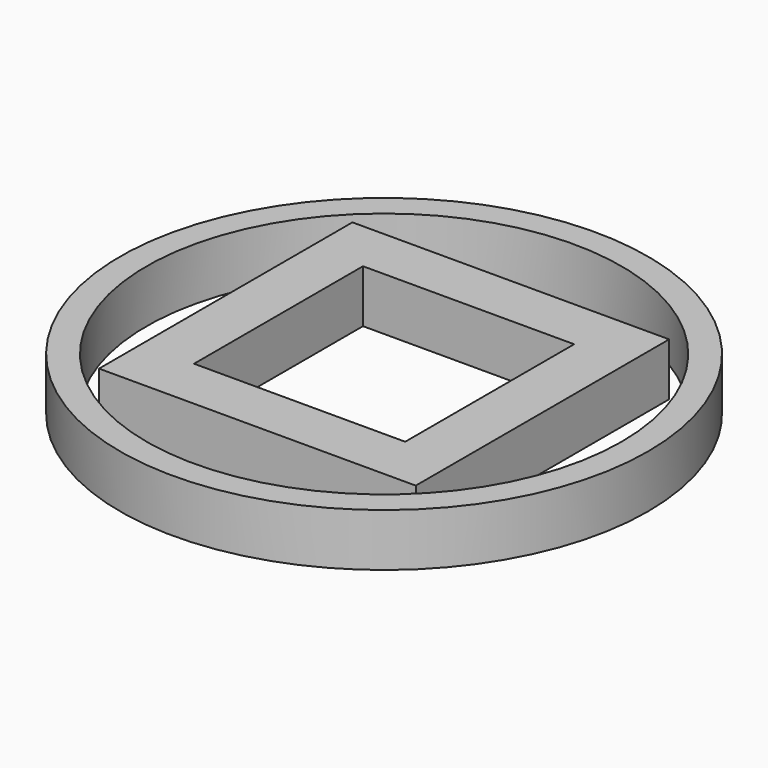
from build123d import *

# Parameters (mm, degrees)
F0_R     = 25
F0_R_2   = 22.5
F1_DEPTH = 5
F2_W     = 30
F2_H     = 30
F2_W_2   = 20
F2_H_2   = 20
F3_DEPTH = 5


# Not quite as in the source:
# - a feature names something its author has since deleted; it is built from what else it names


with BuildPart() as f1:
    # F0 (on Top) → F1 (new body)
    with BuildSketch(Plane.XY):
        Circle(F0_R)
        Circle(F0_R_2, mode=Mode.SUBTRACT)
    extrude(amount=F1_DEPTH)


with BuildPart() as f3:
    # F2 (on face) → F3 (new body)
    with BuildSketch(Plane.XY):
        Rectangle(F2_W, F2_H)
        Rectangle(F2_W_2, F2_H_2, mode=Mode.SUBTRACT)
    extrude(amount=F3_DEPTH)


solid = Compound([f1.part, f3.part])
